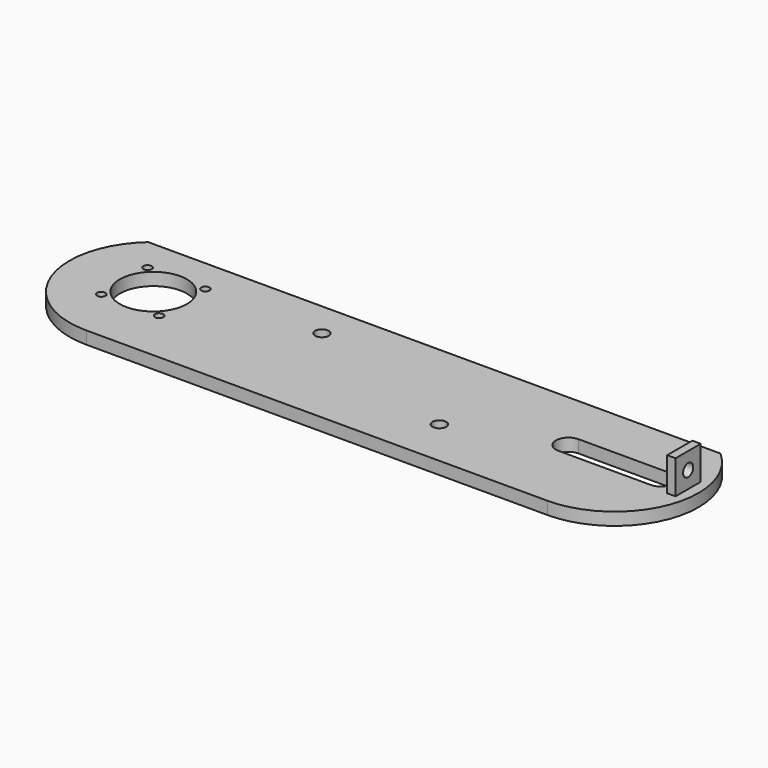
from build123d import *

# Parameters (mm, degrees)
F0_R     = 3.25
F0_R_2   = 16
F1_DEPTH = 6
F2_W     = 4
F2_H     = 15
F3_DEPTH = 16
F4_R     = 3
F5_DEPTH = 25
F6_R     = 2
F7_DEPTH = 25


# Not quite as in the source:
# - ends of sketch curves that miss each other by under 0.0002 mm in the source are joined


with BuildPart() as f1:
    # F0 (on Top) → F1 (new body)
    with BuildSketch(Plane.XY):
        with BuildLine():
            ThreePointArc((110, -105), (147.4165738824, -79.1421355849), (136.4575130484, -34.9999999451))
            Line((136.4575130484, -34.9999999451), (75, -35))
            Line((75, -35), (-75, -35))
            Line((-75, -35), (-136.457514, -35))
            ThreePointArc((-136.457514, -35), (-147.4165737498, -79.1421359357), (-110, -105))
            Line((-110, -105), (-75, -105))
            Line((-75, -105), (75, -105))
            Line((75, -105), (110, -105))
        make_face()
        with Locations((40, -82)):
            Circle(F0_R, mode=Mode.SUBTRACT)
        with Locations((-110, -65)):
            Circle(F0_R_2, mode=Mode.SUBTRACT)
        with Locations((-40, -52)):
            Circle(F0_R, mode=Mode.SUBTRACT)
        with BuildLine():
            Line((88.000112, -59), (131.86291, -59.001567))
            ThreePointArc((131.86291, -59.001567), (137.9996084013, -64.9314505185), (132, -71))
            Line((132, -71), (88, -71))
            ThreePointArc((88, -71), (82.0000000003, -64.999944), (88.000112, -59))
        make_face(mode=Mode.SUBTRACT)
    extrude(amount=F1_DEPTH)

    # F2 (on face) → F3 (join)
    with BuildSketch(Plane.XY.offset(6)):
        with Locations((143, -64.9314505185)):
            Rectangle(F2_W, F2_H)
    extrude(amount=F3_DEPTH)

    # F4 (on face) → F5 (cut)
    with BuildSketch(Plane.YZ.offset(145)):
        with Locations((-64.9314505185, 14)):
            Circle(F4_R)
    extrude(amount=-F5_DEPTH, mode=Mode.SUBTRACT)

    # F6 (on face) → F7 (cut)
    with BuildSketch(Plane.XY.offset(6)):
        with Locations((-123.7885822331, -51.2114177669)):
            Circle(F6_R)
        with Locations((-96.2114177669, -51.2114177669)):
            Circle(F6_R)
        with Locations((-96.2114177669, -78.7885822331)):
            Circle(F6_R)
        with Locations((-123.7885822331, -78.7885822331)):
            Circle(F6_R)
    extrude(amount=-F7_DEPTH, mode=Mode.SUBTRACT)


solid = f1.part
